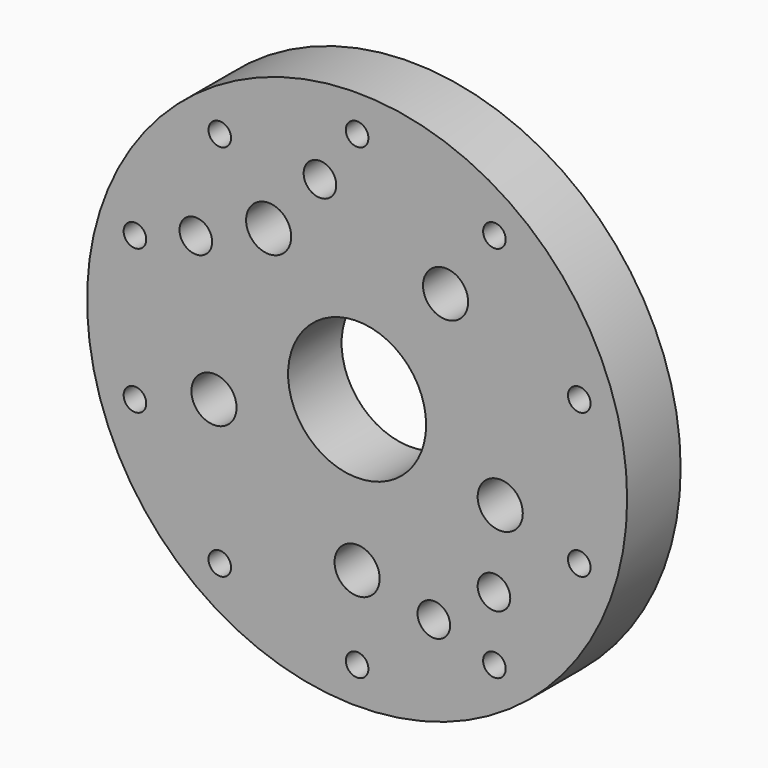
from build123d import *

# Parameters (mm, degrees)
F0_R            = 80.749
F0_R_2          = 4.875
F0_R_3          = 20.6375
F1_DEPTH        = 20
F2_D            = 13.49248
F2_COPIES_COUNT = 5
F3_D            = 6.7564
F3_COPIES_COUNT = 10


# Not quite as in the source:
# - a pattern or mirror of a feature is missing from the dataset's text; its kind, count and spacing are read off the source's solid
# - a feature names something its author has since deleted; it is built from what else it names


with BuildPart() as f1:
    # F0 (on Front) → F1 (new body)
    with BuildSketch(Plane.XZ):
        Circle(F0_R)
        with Locations((-22.9412823532, -50.481680479)):
            Circle(F0_R_2, mode=Mode.SUBTRACT)
        with Locations((-40.9216850532, -37.4181532468)):
            Circle(F0_R_2, mode=Mode.SUBTRACT)
        Circle(F0_R_3, mode=Mode.SUBTRACT)
        with Locations((22.9412823532, -50.481680479)):
            Circle(F0_R_2, mode=Mode.SUBTRACT)
        with Locations((40.9216850532, -37.4181532468)):
            Circle(F0_R_2, mode=Mode.SUBTRACT)
        with Locations((-55.100177293, 6.2187589016)):
            Circle(F0_R_2, mode=Mode.SUBTRACT)
        with Locations((-48.2322745931, 27.3559899762)):
            Circle(F0_R_2, mode=Mode.SUBTRACT)
        with Locations((-11.1125, 54.3250848481)):
            Circle(F0_R_2, mode=Mode.SUBTRACT)
        with Locations((55.100177293, 6.2187589016)):
            Circle(F0_R_2, mode=Mode.SUBTRACT)
        with Locations((48.2322745931, 27.3559899762)):
            Circle(F0_R_2, mode=Mode.SUBTRACT)
        with Locations((11.1125, 54.3250848481)):
            Circle(F0_R_2, mode=Mode.SUBTRACT)
        with Locations((-55.100177293, 6.2187589016)):
            Circle(F0_R_2)
        with Locations((-40.9216850532, -37.4181532468)):
            Circle(F0_R_2)
        with Locations((-22.9412823532, -50.481680479)):
            Circle(F0_R_2)
        with Locations((55.100177293, 6.2187589016)):
            Circle(F0_R_2)
        with Locations((48.2322745931, 27.3559899762)):
            Circle(F0_R_2)
        with Locations((11.1125, 54.3250848481)):
            Circle(F0_R_2)
    extrude(amount=F1_DEPTH)

    # F2 (through all)
    with Locations(Plane(origin=(0, 0, 0), x_dir=(1, 0, 0), z_dir=(0, 1, 0))):
        with Locations((-26.4503363532, -36.4057647469)):
            f2 = Hole(F2_D / 2)

    # F2_copies: F2 ×5 about axis
    f2_copies_axis = Axis((0, 0, 0), (0, 1, 0))
    for i in range(1, F2_COPIES_COUNT):
        add(f2.rotate(f2_copies_axis, i * 360 / F2_COPIES_COUNT), mode=Mode.SUBTRACT)

    # F3 (through all)
    with Locations(Plane(origin=(0, 0, 0), x_dir=(1, 0, 0), z_dir=(0, 1, 0))):
        with Locations((-41.0567998726, -56.5098370571)):
            f3 = Hole(F3_D / 2)

    # F3_copies: F3 ×10 about axis
    f3_copies_axis = Axis((0, 0, 0), (0, 1, 0))
    for i in range(1, F3_COPIES_COUNT):
        add(f3.rotate(f3_copies_axis, i * 360 / F3_COPIES_COUNT), mode=Mode.SUBTRACT)


solid = f1.part
